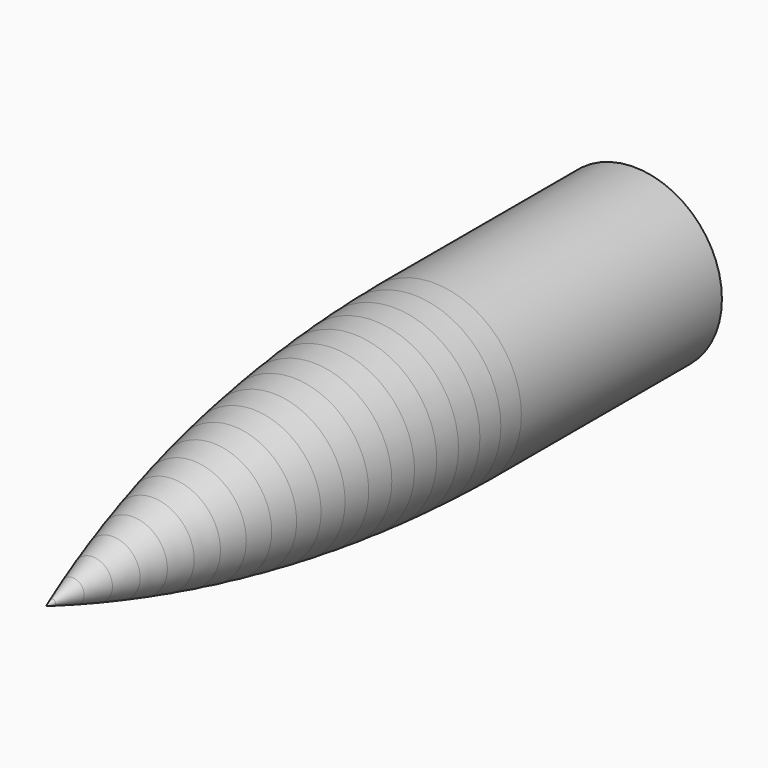
from build123d import *

# Parameters (mm, degrees)
F0_R       = 350
F1_DEPTH   = 100
F1_TAPER   = 1
F1_FACE_R  = 348.2544935072
F2_DEPTH   = 100
F2_TAPER   = 2
F2_FACE_R  = 344.762416558
F3_DEPTH   = 100
F3_TAPER   = 3
F3_FACE_R  = 339.5216386297
F4_DEPTH   = 100
F4_TAPER   = 4
F4_FACE_R  = 332.5289574353
F5_DEPTH   = 100
F5_TAPER   = 5
F5_FACE_R  = 323.7800910828
F6_DEPTH   = 100
F6_TAPER   = 6
F6_FACE_R  = 313.2696675562
F7_DEPTH   = 100
F7_TAPER   = 7
F7_FACE_R  = 300.9912114659
F8_DEPTH   = 100
F8_TAPER   = 8
F8_FACE_R  = 286.9371279957
F9_DEPTH   = 100
F9_TAPER   = 9
F9_FACE_R  = 271.0986839632
F10_DEPTH  = 100
F10_TAPER  = 10
F10_FACE_R = 253.4659858924
F11_DEPTH  = 100
F11_TAPER  = 11
F11_FACE_R = 234.0279549786
F12_DEPTH  = 100
F12_TAPER  = 12
F12_FACE_R = 212.7722988116
F13_DEPTH  = 100
F13_TAPER  = 13
F13_FACE_R = 189.685479699
F14_DEPTH  = 100
F14_TAPER  = 14
F14_FACE_R = 164.7526794147
F15_DEPTH  = 100
F15_TAPER  = 15
F15_FACE_R = 137.9577601716
F16_DEPTH  = 100
F16_TAPER  = 16
F16_FACE_R = 109.2832215957
F17_DEPTH  = 100
F17_TAPER  = 17
F17_FACE_R = 78.7101534499
F18_DEPTH  = 100
F18_TAPER  = 18
F18_FACE_R = 46.2181838266
F19_DEPTH  = 100
F19_TAPER  = 19
F19_FACE_R = 11.7854224976
F21_DEPTH  = 1000


# Not quite as in the source:
# - an extrude whose draft closes it to a point is written as a loft to that point


with BuildPart() as f1:
    # F0 (on Front) → F1 (new body)
    with BuildSketch(Plane.XZ):
        Circle(F0_R)
    extrude(amount=F1_DEPTH, taper=F1_TAPER)

    # F1_face (on face) → F2 (join)
    with BuildSketch(Plane.XZ.offset(100)):
        Circle(F1_FACE_R)
    extrude(amount=F2_DEPTH, taper=F2_TAPER)

    # F2_face (on face) → F3 (join)
    with BuildSketch(Plane.XZ.offset(200)):
        Circle(F2_FACE_R)
    extrude(amount=F3_DEPTH, taper=F3_TAPER)

    # F3_face (on face) → F4 (join)
    with BuildSketch(Plane.XZ.offset(300)):
        Circle(F3_FACE_R)
    extrude(amount=F4_DEPTH, taper=F4_TAPER)

    # F4_face (on face) → F5 (join)
    with BuildSketch(Plane.XZ.offset(400)):
        Circle(F4_FACE_R)
    extrude(amount=F5_DEPTH, taper=F5_TAPER)

    # F5_face (on face) → F6 (join)
    with BuildSketch(Plane.XZ.offset(500)):
        Circle(F5_FACE_R)
    extrude(amount=F6_DEPTH, taper=F6_TAPER)

    # F6_face (on face) → F7 (join)
    with BuildSketch(Plane.XZ.offset(600)):
        Circle(F6_FACE_R)
    extrude(amount=F7_DEPTH, taper=F7_TAPER)

    # F7_face (on face) → F8 (join)
    with BuildSketch(Plane.XZ.offset(700)):
        Circle(F7_FACE_R)
    extrude(amount=F8_DEPTH, taper=F8_TAPER)

    # F8_face (on face) → F9 (join)
    with BuildSketch(Plane.XZ.offset(800)):
        Circle(F8_FACE_R)
    extrude(amount=F9_DEPTH, taper=F9_TAPER)

    # F9_face (on face) → F10 (join)
    with BuildSketch(Plane.XZ.offset(900)):
        Circle(F9_FACE_R)
    extrude(amount=F10_DEPTH, taper=F10_TAPER)

    # F10_face (on face) → F11 (join)
    with BuildSketch(Plane.XZ.offset(1000)):
        Circle(F10_FACE_R)
    extrude(amount=F11_DEPTH, taper=F11_TAPER)

    # F11_face (on face) → F12 (join)
    with BuildSketch(Plane.XZ.offset(1100)):
        Circle(F11_FACE_R)
    extrude(amount=F12_DEPTH, taper=F12_TAPER)

    # F12_face (on face) → F13 (join)
    with BuildSketch(Plane.XZ.offset(1200)):
        Circle(F12_FACE_R)
    extrude(amount=F13_DEPTH, taper=F13_TAPER)

    # F13_face (on face) → F14 (join)
    with BuildSketch(Plane.XZ.offset(1300)):
        Circle(F13_FACE_R)
    extrude(amount=F14_DEPTH, taper=F14_TAPER)

    # F14_face (on face) → F15 (join)
    with BuildSketch(Plane.XZ.offset(1400)):
        Circle(F14_FACE_R)
    extrude(amount=F15_DEPTH, taper=F15_TAPER)

    # F15_face (on face) → F16 (join)
    with BuildSketch(Plane.XZ.offset(1500)):
        Circle(F15_FACE_R)
    extrude(amount=F16_DEPTH, taper=F16_TAPER)

    # F16_face (on face) → F17 (join)
    with BuildSketch(Plane.XZ.offset(1600)):
        Circle(F16_FACE_R)
    extrude(amount=F17_DEPTH, taper=F17_TAPER)

    # F17_face (on face) → F18 (join)
    with BuildSketch(Plane.XZ.offset(1700)):
        Circle(F17_FACE_R)
    extrude(amount=F18_DEPTH, taper=F18_TAPER)

    # F18_face (on face) → F19 (join)
    with BuildSketch(Plane.XZ.offset(1800)):
        Circle(F18_FACE_R)
    extrude(amount=F19_DEPTH, taper=F19_TAPER)

    # F19_face (on face) → F20 section 0
    with BuildSketch(Plane.XZ.offset(1900), mode=Mode.PRIVATE) as f20_s0:
        Circle(F19_FACE_R)
    loft([f20_s0.sketch, Vertex(0, -1932.3801821909, 0)], ruled=True)

    # F21 (add): a face of the model
    f21_faces = [f1.faces().sort_by_distance(p)[0] for p in [
        (0, 0, 0),
    ]]
    extrude(f21_faces, amount=F21_DEPTH)


solid = f1.part
